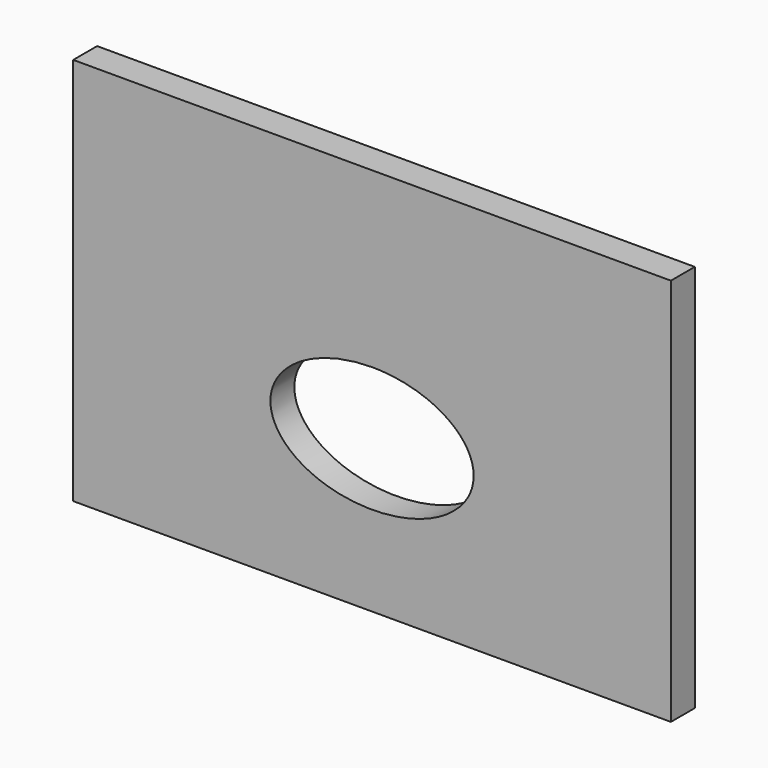
from build123d import *

# Parameters (mm, degrees)
F1_DEPTH = 5


# Not quite as in the source:
# - a feature names something its author has since deleted; it is built from what else it names


with BuildPart() as f1:
    # F0 (on Front) → F1 (new body)
    with BuildSketch(Plane.XZ):
        Polygon((50, 39.5), (0, 39.5), (-50, 39.5), (-50, -25.5), (50, -25.5), align=None)
        with BuildLine():
            add(Edge.make_bspline(
                [(-17, 0), (-17, -25.3492424049), (12.0208152802, -7.4246212025), (41.0416305603, 10.5), (0, 10.5)],
                knots=[0, 0, 0, 2.3561944902, 2.3561944902, 4.7123889804, 4.7123889804, 4.7123889804], degree=2, weights=[1, 0.3826834324, 1, 0.3826834324, 1]))
            add(Edge.make_bspline(
                [(0, 10.5), (-17, 10.5), (-17, 0)],
                knots=[4.7123889804, 4.7123889804, 4.7123889804, 6.2831853072, 6.2831853072, 6.2831853072], degree=2, weights=[1, 0.7071067812, 1]))
        make_face(mode=Mode.SUBTRACT)
    extrude(amount=F1_DEPTH)


solid = f1.part
